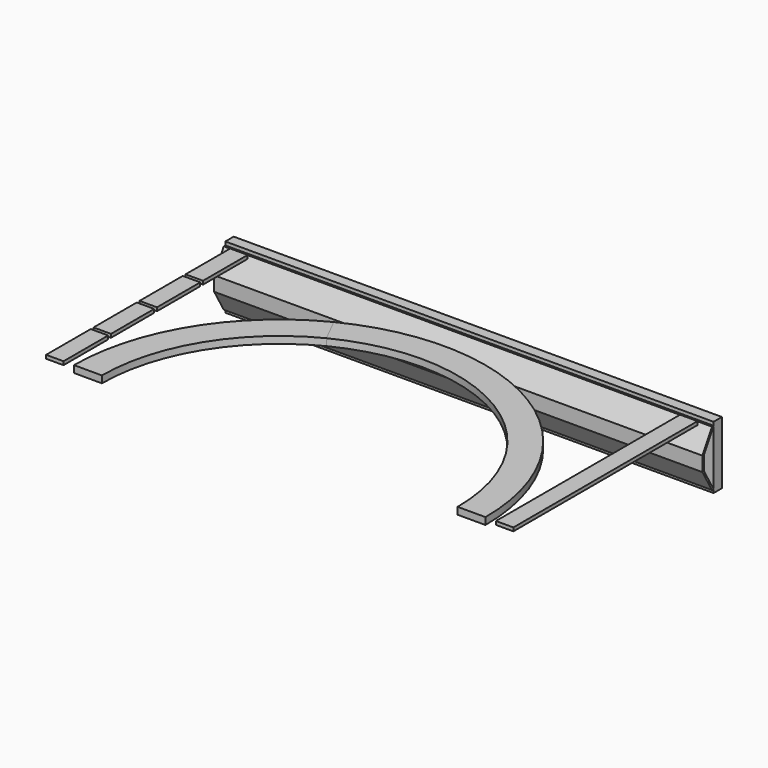
from build123d import *

# Parameters (mm, degrees)
F0_W     = 5
F0_H     = 16
F1_DEPTH = 1
F0_H_2   = 15.5
F2_DEPTH = 2
F0_H_3   = 1
F3_DEPTH = 1
F4_DEPTH = 2
F6_DEPTH = 70


with BuildPart() as f1:
    # F0 (on Top) → F1 (new body)
    with BuildSketch(Plane.XY):
        with Locations((-64.5, 25)):
            Rectangle(F0_W, F0_H)
    extrude(amount=-F1_DEPTH)


with BuildPart() as f1b:
    # F0 (on Top) → F1, piece 2 (new body)
    with BuildSketch(Plane.XY):
        with Locations((-64.5, 8.25)):
            Rectangle(F0_W, F0_H_2)
    extrude(amount=-F1_DEPTH)


with BuildPart() as f1c:
    # F0 (on Top) → F1, piece 3 (new body)
    with BuildSketch(Plane.XY):
        with Locations((-64.5, -8.25)):
            Rectangle(F0_W, F0_H_2)
    extrude(amount=-F1_DEPTH)


with BuildPart() as f1d:
    # F0 (on Top) → F1, piece 4 (new body)
    with BuildSketch(Plane.XY):
        with Locations((-64.5, -25)):
            Rectangle(F0_W, F0_H)
    extrude(amount=-F1_DEPTH)


with BuildPart() as f1e:
    # F0 (on Top) → F1, piece 5 (new body)
    with BuildSketch(Plane.XY):
        with Locations((64.5, 25)):
            Rectangle(F0_W, F0_H)
    extrude(amount=-F1_DEPTH)


with BuildPart() as f1f:
    # F0 (on Top) → F1, piece 6 (new body)
    with BuildSketch(Plane.XY):
        with Locations((64.5, 8.25)):
            Rectangle(F0_W, F0_H_2)
    extrude(amount=-F1_DEPTH)


with BuildPart() as f1g:
    # F0 (on Top) → F1, piece 7 (new body)
    with BuildSketch(Plane.XY):
        with Locations((64.5, -8.25)):
            Rectangle(F0_W, F0_H_2)
    extrude(amount=-F1_DEPTH)


with BuildPart() as f1h:
    # F0 (on Top) → F1, piece 8 (new body)
    with BuildSketch(Plane.XY):
        with Locations((64.5, -25)):
            Rectangle(F0_W, F0_H)
    extrude(amount=-F1_DEPTH)


with BuildPart() as f2:
    # F0 (on Top) → F2 (new body)
    with BuildSketch(Plane.XY):
        with BuildLine():
            Line((-23.0162111194, 12.5110319121), (-26.6265971774, 19.6500173101))
            ThreePointArc((-26.6265971774, 19.6500173101), (-50.2591744534, -2.0966768249), (-59, -33))
            Line((-59, -33), (-51, -33))
            ThreePointArc((-51, -33), (-43.4443711376, -6.2869579334), (-23.0162111194, 12.5110319121))
        make_face()
    extrude(amount=-F2_DEPTH)


with BuildPart() as f3:
    # F0 (on Top) → F3 (new body)
    with BuildSketch(Plane.XY):
        with Locations((64.5, 25)):
            Rectangle(F0_W, F0_H)
        with Locations((64.5, 16.5)):
            Rectangle(F0_W, F0_H_3)
        with Locations((64.5, 8.25)):
            Rectangle(F0_W, F0_H_2)
        with Locations((64.5, 0)):
            Rectangle(F0_W, F0_H_3)
        with Locations((64.5, -8.25)):
            Rectangle(F0_W, F0_H_2)
        with Locations((64.5, -16.5)):
            Rectangle(F0_W, F0_H_3)
        with Locations((64.5, -25)):
            Rectangle(F0_W, F0_H)
    extrude(amount=-F3_DEPTH)


with BuildPart() as f4:
    # F0 (on Top) → F4 (new body)
    with BuildSketch(Plane.XY):
        with BuildLine():
            Line((51, -33), (59, -33))
            ThreePointArc((59, -33), (30.9033231751, 17.2591744534), (-26.6265971774, 19.6500173101))
            Line((-26.6265971774, 19.6500173101), (-23.0162111194, 12.5110319121))
            ThreePointArc((-23.0162111194, 12.5110319121), (26.7130420666, 10.4443711376), (51, -33))
        make_face()
    extrude(amount=-F4_DEPTH)


with BuildPart() as f6:
    # F5 (on Right) → F6 (new body, symmetric)
    with BuildSketch(Plane.YZ):
        Polygon((31.5038475773, -7.0555136271), (35, -1), (34.4226497308, -1), (31.0038475773, -6.9215390309), (31.0038475773, -7.9215390309), align=None)
        Polygon((34.4226497308, -17), (35, -17), (31.5038475773, -10.9444863729), (31.0038475773, -10.0784609691), (31.0038475773, -11.0784609691), align=None)
        Polygon((31.5038475773, -10.9444863729), (31.5038475773, -9), (31.0038475773, -9), (31.0038475773, -10.0784609691), align=None)
        Polygon((31.5038475773, -9), (31.5038475773, -7.0555136271), (31.0038475773, -7.9215390309), (31.0038475773, -9), align=None)
    extrude(amount=F6_DEPTH, both=True)


with BuildPart() as f6b:
    # F5 (on Right) → F6, piece 2 (new body, symmetric)
    with BuildSketch(Plane.YZ):
        Polygon((38, 0), (35, 0), (35, -1), (35, -9), (35, -17), (35, -18), (38, -18), align=None)
    extrude(amount=F6_DEPTH, both=True)


solid = Compound([f1.part, f1b.part, f1c.part, f1d.part, f1e.part, f1f.part, f1g.part, f1h.part, f2.part, f3.part, f4.part, f6.part, f6b.part])
